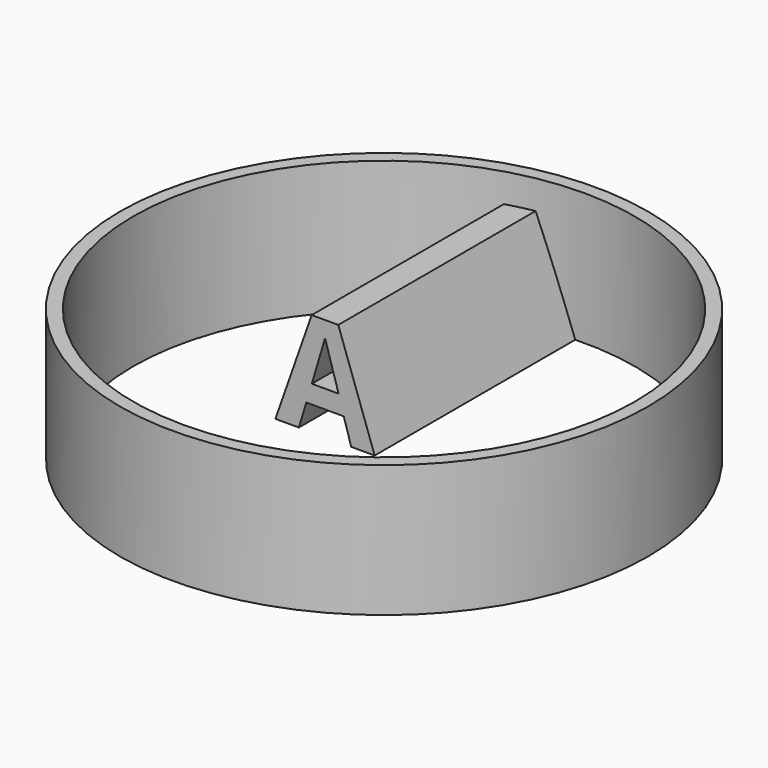
from build123d import *

# Parameters (mm, degrees)
F0_R         = 50.8
F1_DEPTH     = 25.4
F3_D         = 96.52
F4_TEXT_SIZE = 27.6874673242
F5_DEPTH     = 54.102


# Not quite as in the source:
# - Text() gives the source's letters only with a copy of the font that has no kerning and outlines rounded to 1/6400 em; it was checked with that copy


with BuildPart() as f1:
    # F0 (on Top) → F1 (new body)
    with BuildSketch(Plane.XY):
        Circle(F0_R)
    extrude(amount=F1_DEPTH)

    # F3 (through all)
    with Locations(Plane(origin=(0, 0, 0), x_dir=(1, 0, 0), z_dir=(0, 0, -1))):
        with Locations((0, 0)):
            Hole(F3_D / 2)

    # F4 (on Front) → F5 (join)
    with BuildSketch(Plane.XZ):
        with Locations((-20.899711663, 0)):
            Text('A', F4_TEXT_SIZE, font='Open Sans', font_style=FontStyle.BOLD, text_align=(TextAlign.LEFT, TextAlign.BOTTOM))
    extrude(amount=-F5_DEPTH)


solid = f1.part
